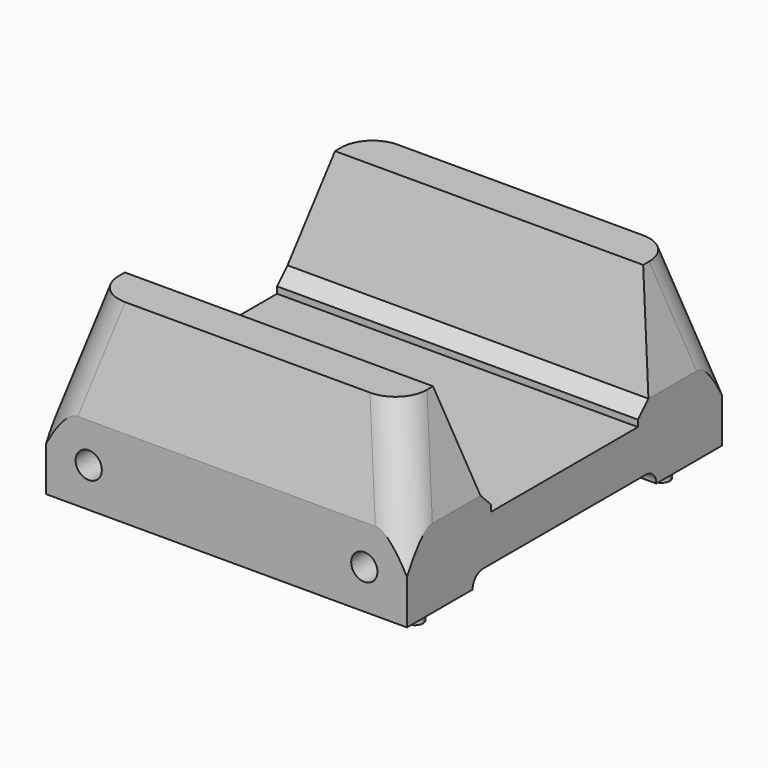
from build123d import *

# Parameters (mm, degrees)
F0_W      = 55
F0_H      = 60
F1_DEPTH  = 12
F2_DEPTH  = 3
F3_W      = 35
F3_H      = 2
F4_DEPTH  = 56.75
F5_R      = 1.99999
F6_R      = 2
F7_DEPTH  = 63.75
F8_W      = 28
F8_H      = 3
F9_DEPTH  = 57.25
F10_SIZE  = 2
F9_FACE_W = 55
F9_FACE_H = 14
F11_DEPTH = 15
F11_TAPER = 15
F12_R     = 5


# Not quite as in the source:
# - a fillet or chamfer is up to 0.001 mm smaller than in the source, because OpenCascade refuses the exact size


with BuildPart() as f1:
    # F0 (on Top) → F1 (new body)
    with BuildSketch(Plane.XY):
        Rectangle(F0_W, F0_H)
        with BuildLine():
            ThreePointArc((-23.5, 22.25), (-24.3838834765, 24.3838834765), (-22.25, 23.5))
            Line((-22.25, 23.5), (22.25, 23.5))
            ThreePointArc((22.25, 23.5), (23.5, 24.75), (24.75, 23.5))
            ThreePointArc((24.75, 23.5), (24.3838834765, 22.6161165235), (23.5, 22.25))
            Line((23.5, 22.25), (23.5, -22.25))
            ThreePointArc((23.5, -22.25), (24.3838834765, -22.6161165235), (24.75, -23.5))
            ThreePointArc((24.75, -23.5), (23.5, -24.75), (22.25, -23.5))
            Line((22.25, -23.5), (-22.25, -23.5))
            ThreePointArc((-22.25, -23.5), (-24.3838834765, -24.3838834765), (-23.5, -22.25))
            Line((-23.5, -22.25), (-23.5, 22.25))
        make_face(mode=Mode.SUBTRACT)
        with BuildLine():
            Line((22.25, 23.5), (-22.25, 23.5))
            ThreePointArc((-22.25, 23.5), (-22.6161165235, 22.6161165235), (-23.5, 22.25))
            Line((-23.5, 22.25), (-23.5, -22.25))
            ThreePointArc((-23.5, -22.25), (-22.6161165235, -22.6161165235), (-22.25, -23.5))
            Line((-22.25, -23.5), (22.25, -23.5))
            ThreePointArc((22.25, -23.5), (22.6161165235, -22.6161165235), (23.5, -22.25))
            Line((23.5, -22.25), (23.5, 22.25))
            ThreePointArc((23.5, 22.25), (22.6161165235, 22.6161165235), (22.25, 23.5))
        make_face()
        with BuildLine():
            Line((-23.5, 22.25), (-23.5, 23.5))
            Line((-23.5, 23.5), (-22.25, 23.5))
            ThreePointArc((-22.25, 23.5), (-24.3838834765, 24.3838834765), (-23.5, 22.25))
        make_face()
        with BuildLine():
            Line((-22.25, 23.5), (-23.5, 23.5))
            Line((-23.5, 23.5), (-23.5, 22.25))
            ThreePointArc((-23.5, 22.25), (-22.6161165235, 22.6161165235), (-22.25, 23.5))
        make_face()
        with BuildLine():
            ThreePointArc((24.75, 23.5), (23.5, 24.75), (22.25, 23.5))
            Line((22.25, 23.5), (23.5, 23.5))
            Line((23.5, 23.5), (23.5, 22.25))
            ThreePointArc((23.5, 22.25), (24.3838834765, 22.6161165235), (24.75, 23.5))
        make_face()
        with BuildLine():
            Line((23.5, 23.5), (22.25, 23.5))
            ThreePointArc((22.25, 23.5), (22.6161165235, 22.6161165235), (23.5, 22.25))
            Line((23.5, 22.25), (23.5, 23.5))
        make_face()
        with BuildLine():
            ThreePointArc((24.75, -23.5), (24.3838834765, -22.6161165235), (23.5, -22.25))
            Line((23.5, -22.25), (23.5, -23.5))
            Line((23.5, -23.5), (22.25, -23.5))
            ThreePointArc((22.25, -23.5), (23.5, -24.75), (24.75, -23.5))
        make_face()
        with BuildLine():
            Line((23.5, -23.5), (23.5, -22.25))
            ThreePointArc((23.5, -22.25), (22.6161165235, -22.6161165235), (22.25, -23.5))
            Line((22.25, -23.5), (23.5, -23.5))
        make_face()
        with BuildLine():
            Line((-23.5, -23.5), (-23.5, -22.25))
            ThreePointArc((-23.5, -22.25), (-24.3838834765, -24.3838834765), (-22.25, -23.5))
            Line((-22.25, -23.5), (-23.5, -23.5))
        make_face()
        with BuildLine():
            ThreePointArc((-22.25, -23.5), (-22.6161165235, -22.6161165235), (-23.5, -22.25))
            Line((-23.5, -22.25), (-23.5, -23.5))
            Line((-23.5, -23.5), (-22.25, -23.5))
        make_face()
    extrude(amount=F1_DEPTH)

    # F0 (on Top) → F2 (join)
    with BuildSketch(Plane.XY):
        with BuildLine():
            Line((-23.5, 22.25), (-23.5, 23.5))
            Line((-23.5, 23.5), (-22.25, 23.5))
            ThreePointArc((-22.25, 23.5), (-24.3838834765, 24.3838834765), (-23.5, 22.25))
        make_face()
        with BuildLine():
            Line((-22.25, 23.5), (-23.5, 23.5))
            Line((-23.5, 23.5), (-23.5, 22.25))
            ThreePointArc((-23.5, 22.25), (-22.6161165235, 22.6161165235), (-22.25, 23.5))
        make_face()
        with BuildLine():
            Line((-23.5, -23.5), (-23.5, -22.25))
            ThreePointArc((-23.5, -22.25), (-24.3838834765, -24.3838834765), (-22.25, -23.5))
            Line((-22.25, -23.5), (-23.5, -23.5))
        make_face()
        with BuildLine():
            ThreePointArc((-22.25, -23.5), (-22.6161165235, -22.6161165235), (-23.5, -22.25))
            Line((-23.5, -22.25), (-23.5, -23.5))
            Line((-23.5, -23.5), (-22.25, -23.5))
        make_face()
        with BuildLine():
            ThreePointArc((24.75, -23.5), (24.3838834765, -22.6161165235), (23.5, -22.25))
            Line((23.5, -22.25), (23.5, -23.5))
            Line((23.5, -23.5), (22.25, -23.5))
            ThreePointArc((22.25, -23.5), (23.5, -24.75), (24.75, -23.5))
        make_face()
        with BuildLine():
            Line((23.5, -23.5), (23.5, -22.25))
            ThreePointArc((23.5, -22.25), (22.6161165235, -22.6161165235), (22.25, -23.5))
            Line((22.25, -23.5), (23.5, -23.5))
        make_face()
        with BuildLine():
            ThreePointArc((24.75, 23.5), (23.5, 24.75), (22.25, 23.5))
            Line((22.25, 23.5), (23.5, 23.5))
            Line((23.5, 23.5), (23.5, 22.25))
            ThreePointArc((23.5, 22.25), (24.3838834765, 22.6161165235), (24.75, 23.5))
        make_face()
        with BuildLine():
            Line((23.5, 23.5), (22.25, 23.5))
            ThreePointArc((22.25, 23.5), (22.6161165235, 22.6161165235), (23.5, 22.25))
            Line((23.5, 22.25), (23.5, 23.5))
        make_face()
    extrude(amount=-F2_DEPTH)

    # F3 (on face) → F4 (cut)
    with BuildSketch(Plane.YZ.offset(27.5)):
        with Locations((0, 1)):
            Rectangle(F3_W, F3_H)
    extrude(amount=-F4_DEPTH, mode=Mode.SUBTRACT)

    # F5 (radius 2 in the source; OpenCascade refuses exactly that, so slightly less here)
    f5_edges = [f1.edges().sort_by_distance(p)[0] for p in [
        (0, -17.5, 2),
        (0, 17.5, 2),
    ]]
    fillet(f5_edges, radius=F5_R)

    # F6 (on face) → F7 (cut)
    with BuildSketch(Plane(origin=(0, 30, 0), x_dir=(-1, 0, 0), z_dir=(0, 1, 0))):
        with Locations((-21, 6)):
            Circle(F6_R)
        with Locations((21, 6)):
            Circle(F6_R)
    extrude(amount=-F7_DEPTH, mode=Mode.SUBTRACT)

    # F8 (on face) → F9 (cut)
    with BuildSketch(Plane(origin=(-27.5, 0, 0), x_dir=(0, -1, 0), z_dir=(-1, 0, 0))):
        with Locations((0, 10.5)):
            Rectangle(F8_W, F8_H)
    extrude(amount=-F9_DEPTH, mode=Mode.SUBTRACT)

    # F10
    f10_edges = [f1.edges().sort_by_distance(p)[0] for p in [
        (0, -14, 12),
        (0, 14, 12),
    ]]
    chamfer(f10_edges, length=F10_SIZE)

    # F9_face (on face) → F11 (join)
    with BuildSketch(Plane(origin=(0, 23, 12), x_dir=(1, 0, 0), z_dir=(0, 0, 1))):
        Rectangle(F9_FACE_W, F9_FACE_H)
        with Locations((0, -46)):
            Rectangle(F9_FACE_W, F9_FACE_H)
    extrude(amount=F11_DEPTH, taper=F11_TAPER)

    # F12
    f12_edges = [f1.edges().sort_by_distance(p)[0] for p in [
        (-25.490381, 27.990381, 19.5),
        (25.490381, 27.990381, 19.5),
        (-25.490381, -27.990381, 19.5),
        (25.490381, -27.990381, 19.5),
    ]]
    fillet(f12_edges, radius=F12_R)


solid = f1.part
